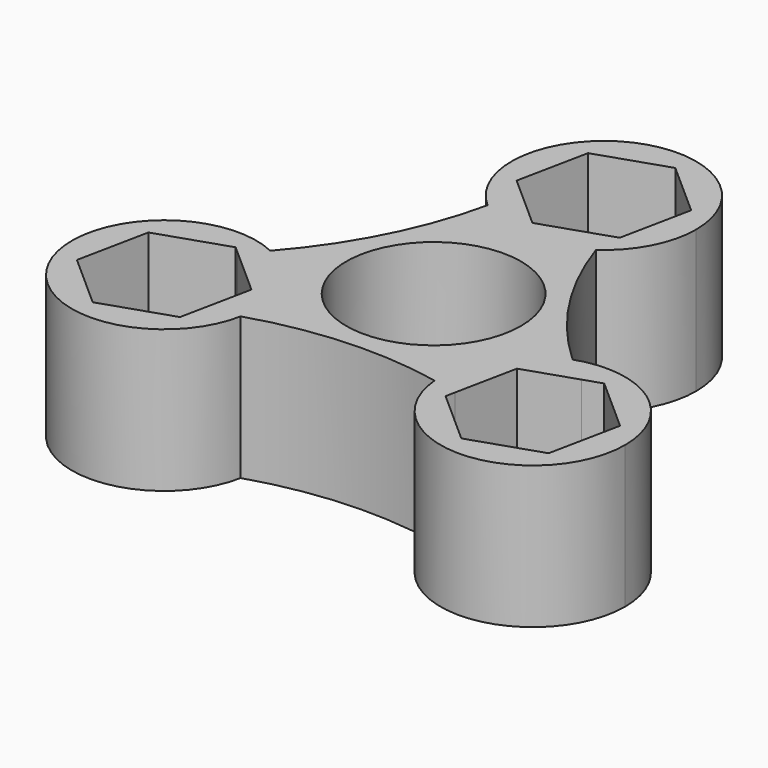
from build123d import *

# Parameters (mm, degrees)
F0_R     = 15.5998218224
F1_DEPTH = 25.4


# Not quite as in the source:
# - a feature of the source that left no trace in its solid (it failed there, or was rolled back) is left out


with BuildPart() as f1:
    # F0 (on Top) → F1 (new body)
    with BuildSketch(Plane.XY):
        with BuildLine():
            Line((-9.7679234278, 31.6427110991), (-12.2910759721, 33.8783473239))
            Line((-12.2910759721, 33.8783473239), (-9.6983198699, 46.5739309325))
            Line((-9.6983198699, 46.5739309325), (2.5927561023, 50.6763300865))
            Line((2.5927561023, 50.6763300865), (12.2910759721, 42.0831456318))
            Line((12.2910759721, 42.0831456318), (9.6983198699, 29.3875620231))
            Line((9.6983198699, 29.3875620231), (8.1033290175, 28.8552010534))
            ThreePointArc((8.1033290175, 28.8552010534), (8.7164308394, 26.6457057993), (9.4057371171, 24.4587855955))
            ThreePointArc((9.4057371171, 24.4587855955), (14.5985992918, 30.3523642419), (16.4715304941, 37.9807464778))
            ThreePointArc((16.4715304941, 37.9807464778), (-6.8274979981, 52.9706293294), (-10.8114943571, 25.5540451221))
            ThreePointArc((-10.8114943571, 25.5540451221), (-10.2185999519, 28.5861903467), (-9.7679234278, 31.6427110991))
        make_face()
        with BuildLine():
            Line((-2.5927561023, 25.2851628692), (-9.7679234278, 31.6427110991))
            ThreePointArc((-9.7679234278, 31.6427110991), (-10.2185999519, 28.5861903467), (-10.8114943571, 25.5540451221))
            ThreePointArc((-10.8114943571, 25.5540451221), (-0.8910312632, 21.5333339121), (9.4057371171, 24.4587855955))
            ThreePointArc((9.4057371171, 24.4587855955), (8.7164308394, 26.6457057993), (8.1033290175, 28.8552010534))
            Line((8.1033290175, 28.8552010534), (-2.5927561023, 25.2851628692))
        make_face()
        with BuildLine():
            ThreePointArc((9.4057371171, 24.4587855955), (-0.8910312632, 21.5333339121), (-10.8114943571, 25.5540451221))
            ThreePointArc((-10.8114943571, 25.5540451221), (-16.4556801257, 9.772653233), (-25.88479823, -4.083785513))
            ThreePointArc((-25.88479823, -4.083785513), (-27.4340735437, -5.7742023624), (-29.0410016523, -7.4099117424))
            Line((-29.0410016523, -7.4099117424), (-20.6012153324, -14.887974085))
            Line((-20.6012153324, -14.887974085), (-22.5194299425, -24.2806253802))
            ThreePointArc((-22.5194299425, -24.2806253802), (-19.6470670617, -23.1426623228), (-16.7247050666, -22.1400513271))
            ThreePointArc((-16.7247050666, -22.1400513271), (-0.2355258993, -19.1373636419), (16.4790611129, -20.3750000825))
            ThreePointArc((16.4790611129, -20.3750000825), (19.0939298277, -9.9950112466), (27.5361994237, -3.4139937949))
            ThreePointArc((27.5361994237, -3.4139937949), (16.691206025, 9.3647104089), (9.4057371171, 24.4587855955))
        make_face()
        Circle(F0_R, mode=Mode.SUBTRACT)
        with BuildLine():
            ThreePointArc((-29.0410016523, -7.4099117424), (-27.4340735437, -5.7742023624), (-25.88479823, -4.083785513))
            ThreePointArc((-25.88479823, -4.083785513), (-47.5816840445, -26.4424238123), (-16.7247050666, -22.1400513271))
            ThreePointArc((-16.7247050666, -22.1400513271), (-19.6470670617, -23.1426623228), (-22.5194299425, -24.2806253802))
            Line((-22.5194299425, -24.2806253802), (-23.1939714347, -27.5835576936))
            Line((-23.1939714347, -27.5835576936), (-35.4850474068, -31.6859568476))
            Line((-35.4850474068, -31.6859568476), (-45.1833672766, -23.0927723929))
            Line((-45.1833672766, -23.0927723929), (-42.5906111744, -10.3971887842))
            Line((-42.5906111744, -10.3971887842), (-30.2995352023, -6.2947896303))
            Line((-30.2995352023, -6.2947896303), (-29.0410016523, -7.4099117424))
        make_face()
        with BuildLine():
            ThreePointArc((49.3638217986, -18.9903732389), (42.4601616546, -5.5826451025), (27.5361994237, -3.4139937949))
            ThreePointArc((27.5361994237, -3.4139937949), (29.8656670136, -5.4435280239), (32.2873533703, -7.3620857189))
            Line((32.2873533703, -7.3620857189), (35.4850474068, -6.2947896303))
            Line((35.4850474068, -6.2947896303), (45.1833672766, -14.887974085))
            Line((45.1833672766, -14.887974085), (42.5906111744, -27.5835576936))
            Line((42.5906111744, -27.5835576936), (30.2995352023, -31.6859568476))
            Line((30.2995352023, -31.6859568476), (20.6012153324, -23.0927723929))
            Line((20.6012153324, -23.0927723929), (20.9376726348, -21.4452893111))
            ThreePointArc((20.9376726348, -21.4452893111), (18.7176427043, -20.8715034369), (16.4790611129, -20.3750000825))
            ThreePointArc((16.4790611129, -20.3750000825), (33.5852181443, -35.4473222032), (49.3638217986, -18.9903732389))
        make_face()
        with BuildLine():
            ThreePointArc((32.2873533703, -7.3620857189), (29.8656670136, -5.4435280239), (27.5361994237, -3.4139937949))
            ThreePointArc((27.5361994237, -3.4139937949), (19.0939298277, -9.9950112466), (16.4790611129, -20.3750000825))
            ThreePointArc((16.4790611129, -20.3750000825), (18.7176427043, -20.8715034369), (20.9376726348, -21.4452893111))
            Line((20.9376726348, -21.4452893111), (23.1939714347, -10.3971887842))
            Line((23.1939714347, -10.3971887842), (32.2873533703, -7.3620857189))
        make_face()
    extrude(amount=F1_DEPTH)


solid = f1.part
